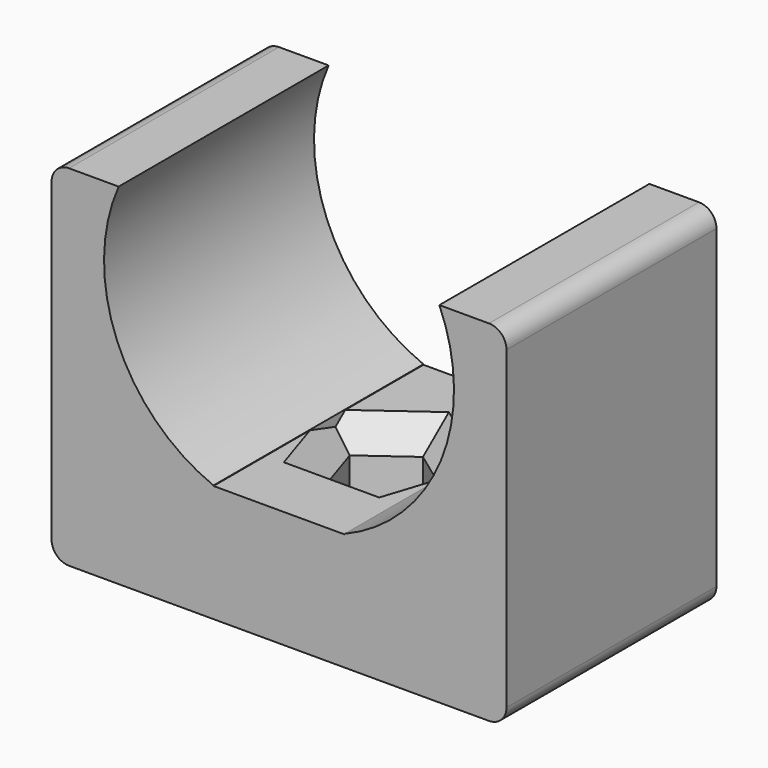
from build123d import *

# Parameters (mm, degrees)
F1_DEPTH     = 15
F3_DEPTH     = 8
F4_W         = 7.4894965633
F4_H         = 15
F5_DEPTH     = 8
F6_DEPTH     = 6.7
F7_T4_DEPTH  = 10.9844903399
F7_T10_DEPTH = 10.9844903399
F7_T16_DEPTH = 10.9844903399
F7_T23_DEPTH = 10.9844903399
F7_T29_DEPTH = 10.9844903399
F7_T37_DEPTH = 10.9844903399
F7_T41_DEPTH = 10.9844903399
F7_T48_DEPTH = 10.9844903399
F7_T53_DEPTH = 10.9844903399
F7_T61_DEPTH = 10.9844903399
F7_T66_DEPTH = 10.9844903399
F7_T74_DEPTH = 10.9844903399
F7_T79_DEPTH = 10.9844903399
F7_T86_DEPTH = 10.9844903399
F7_T91_DEPTH = 10.9844903399
F8_R         = 1


# Not quite as in the source:
# - a fillet or chamfer that OpenCascade refuses, or shapes differently, is made with other operations: its cross-section is extruded or revolved along the edge and cut away or added
# - a feature names something its author has since deleted; it is built from what else it names


with BuildPart() as f1:
    # F0 (on Front) → F1 (new body)
    with BuildSketch(Plane.XZ):
        with BuildLine():
            Line((-11.4096143179, 21.3526541356), (-15.244462928, 21.3526541356))
            Line((-15.244462928, 21.3526541356), (-15.244462928, 1.3526541356))
            Line((-15.244462928, 1.3526541356), (10.755537072, 1.3526541356))
            Line((10.755537072, 1.3526541356), (10.755537072, 21.3526541356))
            Line((10.755537072, 21.3526541356), (6.9206884619, 21.3526541356))
            ThreePointArc((6.9206884619, 21.3526541356), (-2.244462928, 7.3526541356), (-11.4096143179, 21.3526541356))
        make_face()
    extrude(amount=F1_DEPTH)

    # F2 (on face) → F3 (cut)
    with BuildSketch(Plane(origin=(0, 0, 1.3526541356), x_dir=(1, 0, 0), z_dir=(0, 0, -1))):
        Polygon((-0.60974224, 9.75), (-3.879183616, 9.75), (-4.8894965633, 6.6405764747), (-2.244462928, 4.7188470506), (0.4005707074, 6.6405764747), align=None)
    extrude(amount=-F3_DEPTH, mode=Mode.SUBTRACT)

    # F4 (on face) → F5 (cut)
    with BuildSketch(Plane(origin=(0, 0, 1.3526541356), x_dir=(1, 0, 0), z_dir=(0, 0, -1))):
        with Locations((-2.2447482816, 7.5)):
            Rectangle(F4_W, F4_H)
        Polygon((0.4005707074, 6.6405764747), (-2.244462928, 4.7188470506), (-4.8894965633, 6.6405764747), (-3.879183616, 9.75), (-0.60974224, 9.75), align=None, mode=Mode.SUBTRACT)
    extrude(amount=-F5_DEPTH, mode=Mode.SUBTRACT)

    # F4 (on face) → F6 (join)
    with BuildSketch(Plane(origin=(0, 0, 1.3526541356), x_dir=(1, 0, 0), z_dir=(0, 0, -1))):
        with Locations((-2.2447482816, 7.5)):
            Rectangle(F4_W, F4_H)
        Polygon((0.4005707074, 6.6405764747), (-2.244462928, 4.7188470506), (-4.8894965633, 6.6405764747), (-3.879183616, 9.75), (-0.60974224, 9.75), align=None, mode=Mode.SUBTRACT)
    extrude(amount=-F6_DEPTH)

    # F7: chamfer of 1.5 on 5 edges, made by hand


with BuildPart() as f7_tool2:
    # F7_s3 → F7_t4 (new body)
    with BuildSketch(Plane(origin=(-0.5921623143, -0.4302311048, 0), x_dir=(0, 0, 1), z_dir=(-0.8090169944, -0.5877852523, 0))):
        Polygon((8.0526541356, -0.9983652494), (6.5526541356, -2.4983652494), (8.0526541356, -2.4983652494), align=None)
    extrude(amount=F7_T4_DEPTH)

    split(bisect_by=Plane(origin=(-3.0193879884, -4.1558310382, 0), x_dir=(0, 0, 1), z_dir=(-0.5877852523, -0.8090169944, 0)), keep=Keep.TOP)

    split(bisect_by=Plane(origin=(-6.3742076477, -2.0711056126, 0), x_dir=(0, 0, 1), z_dir=(0.9510565163, 0.3090169944, 0)), keep=Keep.TOP)


with BuildPart() as f1_1:
    add(f1.part)

    # F7_t1: cut F7_tool2
    add(f7_tool2.part, mode=Mode.SUBTRACT)


with BuildPart() as f7_tool8:
    # F7_s9 → F7_t10 (new body)
    with BuildSketch(Plane(origin=(6.5407615579, -4.7521414374, 0), x_dir=(0, 0, 1), z_dir=(-0.8090169944, 0.5877852523, 0))):
        Polygon((8.0526541356, -3.6368896662), (6.5526541356, -5.1368896662), (8.0526541356, -5.1368896662), align=None)
    extrude(amount=F7_T10_DEPTH)

    split(bisect_by=Plane(origin=(2.3139360678, -0.7518434043, 0), x_dir=(0, 0, 1), z_dir=(-0.9510565163, 0.3090169944, 0)), keep=Keep.TOP)

    split(bisect_by=Plane(origin=(1.4685022485, -2.021219945, 0), x_dir=(0, 0, 1), z_dir=(0.5877852523, -0.8090169944, 0)), keep=Keep.TOP)


with BuildPart() as f1_2:
    add(f1_1.part)

    # F7_t7: cut F7_tool8
    add(f7_tool8.part, mode=Mode.SUBTRACT)


with BuildPart() as f7_tool14:
    # F7_s15 → F7_t16 (new body)
    with BuildSketch(Plane(origin=(-4.1157189289, -12.6668803911, 0), x_dir=(0, 0, 1), z_dir=(0.3090169944, 0.9510565163, 0))):
        Polygon((8.0526541356, 3.9330163646), (6.5526541356, 2.4330163646), (8.0526541356, 2.4330163646), align=None)
    extrude(amount=F7_T16_DEPTH)

    split(bisect_by=Plane.XZ.offset(9.75), keep=Keep.BOTTOM)

    split(bisect_by=Plane(origin=(-3.0193879884, -4.1558310382, 0), x_dir=(0, 0, 1), z_dir=(-0.5877852523, -0.8090169944, 0)), keep=Keep.TOP)

    split(bisect_by=Plane.YZ.offset(1.5), keep=Keep.BOTTOM)


with BuildPart() as f1_3:
    add(f1_2.part)

    # F7_t13: cut F7_tool14
    add(f7_tool14.part, mode=Mode.SUBTRACT)


with BuildPart() as f7_tool21:
    # F7_s22 → F7_t23 (new body)
    with BuildSketch(Plane.YZ.offset(-7.7367080979)):
        Polygon((-9.75, 6.5526541356), (-11.25, 8.0526541356), (-9.75, 8.0526541356), align=None)
    extrude(amount=F7_T23_DEPTH)

    split(bisect_by=Plane(origin=(2.3139360678, -0.7518434043, 0), x_dir=(0, 0, 1), z_dir=(-0.9510565163, 0.3090169944, 0)), keep=Keep.TOP)

    split(bisect_by=Plane(origin=(-6.3742076477, -2.0711056126, 0), x_dir=(0, 0, 1), z_dir=(0.9510565163, 0.3090169944, 0)), keep=Keep.TOP)


with BuildPart() as f1_4:
    add(f1_3.part)

    # F7_t20: cut F7_tool21
    add(f7_tool21.part, mode=Mode.SUBTRACT)


with BuildPart() as f7_tool27:
    # F7_s28 → F7_t29 (new body)
    with BuildSketch(Plane(origin=(0.2926704633, -0.9007470667, 0), x_dir=(0, 0, 1), z_dir=(0.3090169944, -0.9510565163, 0))):
        Polygon((8.0526541356, 8.202238551), (6.5526541356, 6.702238551), (8.0526541356, 6.702238551), align=None)
    extrude(amount=F7_T29_DEPTH)

    split(bisect_by=Plane.XZ.offset(9.75), keep=Keep.BOTTOM)

    split(bisect_by=Plane.YZ.offset(-5.9894965633), keep=Keep.TOP)

    split(bisect_by=Plane(origin=(1.4685022485, -2.021219945, 0), x_dir=(0, 0, 1), z_dir=(0.5877852523, -0.8090169944, 0)), keep=Keep.TOP)


with BuildPart() as f1_5:
    add(f1_4.part)

    # F7_t26: cut F7_tool27
    add(f7_tool27.part, mode=Mode.SUBTRACT)


with BuildPart() as f7_tool35:
    # F7_s36 → F7_t37 (new body)
    with BuildSketch(Plane(origin=(6.5407615579, -4.7521414374, 0), x_dir=(0, 0, 1), z_dir=(-0.8090169944, 0.5877852523, 0))):
        Polygon((8.0526541356, -3.6368896662), (6.5526541356, -5.1368896662), (8.0526541356, -5.1368896662), align=None)
    extrude(amount=F7_T37_DEPTH)

    split(bisect_by=Plane(origin=(1.4685022485, -2.021219945, 0), x_dir=(0, 0, 1), z_dir=(-0.5877852523, 0.8090169944, 0)), keep=Keep.TOP)


with BuildPart() as f7_tool39:
    # F7_s40 → F7_t41 (new body)
    with BuildSketch(Plane(origin=(-0.5921623143, -0.4302311048, 0), x_dir=(0, 0, 1), z_dir=(-0.8090169944, -0.5877852523, 0))):
        Polygon((8.0526541356, -0.9983652494), (6.5526541356, -2.4983652494), (8.0526541356, -2.4983652494), align=None)
    extrude(amount=F7_T41_DEPTH)

    split(bisect_by=Plane(origin=(-3.0193879884, -4.1558310382, 0), x_dir=(0, 0, 1), z_dir=(0.5877852523, 0.8090169944, 0)), keep=Keep.TOP)


with BuildPart() as f7_tool35_1:
    add(f7_tool35.part)

    # F7_t43: intersect F7_tool39
    add(f7_tool39.part, mode=Mode.INTERSECT)


with BuildPart() as f1_6:
    add(f1_5.part)

    # F7_t33: cut F7_tool35
    add(f7_tool35_1.part, mode=Mode.SUBTRACT)


with BuildPart() as f7_tool46:
    # F7_s47 → F7_t48 (new body)
    with BuildSketch(Plane(origin=(-0.5921623143, -0.4302311048, 0), x_dir=(0, 0, 1), z_dir=(-0.8090169944, -0.5877852523, 0))):
        Polygon((8.0526541356, -0.9983652494), (6.5526541356, -2.4983652494), (8.0526541356, -2.4983652494), align=None)
    extrude(amount=F7_T48_DEPTH)

    split(bisect_by=Plane.YZ.offset(-5.9894965633), keep=Keep.TOP)

    split(bisect_by=Plane(origin=(-6.3742076477, -2.0711056126, 0), x_dir=(0, 0, 1), z_dir=(-0.9510565163, -0.3090169944, 0)), keep=Keep.TOP)


with BuildPart() as f7_tool51:
    # F7_s52 → F7_t53 (new body)
    with BuildSketch(Plane(origin=(0.2926704633, -0.9007470667, 0), x_dir=(0, 0, 1), z_dir=(0.3090169944, -0.9510565163, 0))):
        Polygon((8.0526541356, 8.202238551), (6.5526541356, 6.702238551), (8.0526541356, 6.702238551), align=None)
    extrude(amount=F7_T53_DEPTH)

    split(bisect_by=Plane.YZ.offset(-5.9894965633), keep=Keep.TOP)

    split(bisect_by=Plane(origin=(1.4685022485, -2.021219945, 0), x_dir=(0, 0, 1), z_dir=(-0.5877852523, 0.8090169944, 0)), keep=Keep.TOP)


with BuildPart() as f7_tool46_1:
    add(f7_tool46.part)

    # F7_t56: intersect F7_tool51
    add(f7_tool51.part, mode=Mode.INTERSECT)


with BuildPart() as f1_7:
    add(f1_6.part)

    # F7_t44: cut F7_tool46
    add(f7_tool46_1.part, mode=Mode.SUBTRACT)


with BuildPart() as f7_tool59:
    # F7_s60 → F7_t61 (new body)
    with BuildSketch(Plane(origin=(-4.1157189289, -12.6668803911, 0), x_dir=(0, 0, 1), z_dir=(0.3090169944, 0.9510565163, 0))):
        Polygon((8.0526541356, 3.9330163646), (6.5526541356, 2.4330163646), (8.0526541356, 2.4330163646), align=None)
    extrude(amount=F7_T61_DEPTH)

    split(bisect_by=Plane(origin=(-3.0193879884, -4.1558310382, 0), x_dir=(0, 0, 1), z_dir=(0.5877852523, 0.8090169944, 0)), keep=Keep.TOP)

    split(bisect_by=Plane.YZ.offset(1.5), keep=Keep.BOTTOM)


with BuildPart() as f7_tool64:
    # F7_s65 → F7_t66 (new body)
    with BuildSketch(Plane(origin=(6.5407615579, -4.7521414374, 0), x_dir=(0, 0, 1), z_dir=(-0.8090169944, 0.5877852523, 0))):
        Polygon((8.0526541356, -3.6368896662), (6.5526541356, -5.1368896662), (8.0526541356, -5.1368896662), align=None)
    extrude(amount=F7_T66_DEPTH)

    split(bisect_by=Plane(origin=(2.3139360678, -0.7518434043, 0), x_dir=(0, 0, 1), z_dir=(0.9510565163, -0.3090169944, 0)), keep=Keep.TOP)

    split(bisect_by=Plane.YZ.offset(1.5), keep=Keep.BOTTOM)


with BuildPart() as f7_tool59_1:
    add(f7_tool59.part)

    # F7_t69: intersect F7_tool64
    add(f7_tool64.part, mode=Mode.INTERSECT)


with BuildPart() as f1_8:
    add(f1_7.part)

    # F7_t57: cut F7_tool59
    add(f7_tool59_1.part, mode=Mode.SUBTRACT)


with BuildPart() as f7_tool72:
    # F7_s73 → F7_t74 (new body)
    with BuildSketch(Plane.YZ.offset(-7.7367080979)):
        Polygon((-9.75, 6.5526541356), (-11.25, 8.0526541356), (-9.75, 8.0526541356), align=None)
    extrude(amount=F7_T74_DEPTH)

    split(bisect_by=Plane(origin=(2.3139360678, -0.7518434043, 0), x_dir=(0, 0, 1), z_dir=(0.9510565163, -0.3090169944, 0)), keep=Keep.TOP)

    split(bisect_by=Plane.YZ.offset(1.5), keep=Keep.BOTTOM)


with BuildPart() as f7_tool77:
    # F7_s78 → F7_t79 (new body)
    with BuildSketch(Plane(origin=(-4.1157189289, -12.6668803911, 0), x_dir=(0, 0, 1), z_dir=(0.3090169944, 0.9510565163, 0))):
        Polygon((8.0526541356, 3.9330163646), (6.5526541356, 2.4330163646), (8.0526541356, 2.4330163646), align=None)
    extrude(amount=F7_T79_DEPTH)

    split(bisect_by=Plane.XZ.offset(9.75), keep=Keep.TOP)


with BuildPart() as f7_tool72_1:
    add(f7_tool72.part)

    # F7_t81: intersect F7_tool77
    add(f7_tool77.part, mode=Mode.INTERSECT)


with BuildPart() as f1_9:
    add(f1_8.part)

    # F7_t70: cut F7_tool72
    add(f7_tool72_1.part, mode=Mode.SUBTRACT)


with BuildPart() as f7_tool84:
    # F7_s85 → F7_t86 (new body)
    with BuildSketch(Plane.YZ.offset(-7.7367080979)):
        Polygon((-9.75, 6.5526541356), (-11.25, 8.0526541356), (-9.75, 8.0526541356), align=None)
    extrude(amount=F7_T86_DEPTH)

    split(bisect_by=Plane.YZ.offset(-5.9894965633), keep=Keep.TOP)

    split(bisect_by=Plane(origin=(-6.3742076477, -2.0711056126, 0), x_dir=(0, 0, 1), z_dir=(-0.9510565163, -0.3090169944, 0)), keep=Keep.TOP)


with BuildPart() as f7_tool89:
    # F7_s90 → F7_t91 (new body)
    with BuildSketch(Plane(origin=(0.2926704633, -0.9007470667, 0), x_dir=(0, 0, 1), z_dir=(0.3090169944, -0.9510565163, 0))):
        Polygon((8.0526541356, 8.202238551), (6.5526541356, 6.702238551), (8.0526541356, 6.702238551), align=None)
    extrude(amount=F7_T91_DEPTH)

    split(bisect_by=Plane.XZ.offset(9.75), keep=Keep.TOP)


with BuildPart() as f7_tool84_1:
    add(f7_tool84.part)

    # F7_t93: intersect F7_tool89
    add(f7_tool89.part, mode=Mode.INTERSECT)


with BuildPart() as f1_10:
    add(f1_9.part)

    # F7_t82: cut F7_tool84
    add(f7_tool84_1.part, mode=Mode.SUBTRACT)

    # F8
    f8_edges = [f1_10.edges().sort_by_distance(p)[0] for p in [
        (-15.244463, -7.5, 21.352654),
        (10.755537, -7.5, 21.352654),
        (10.755537, -7.5, 1.352654),
        (-15.244463, -7.5, 1.352654),
    ]]
    fillet(f8_edges, radius=F8_R)


solid = f1_10.part
